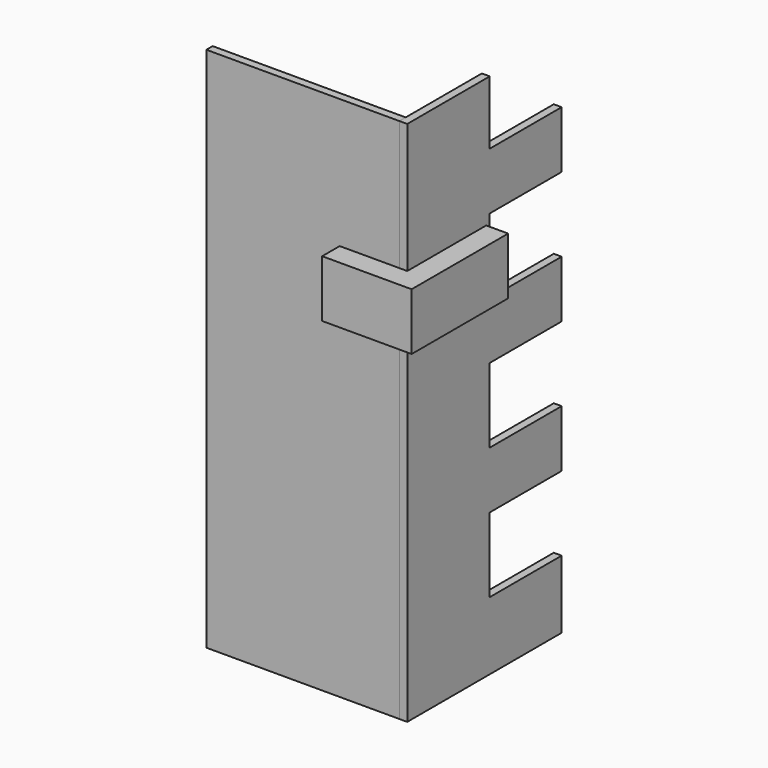
from build123d import *

# Parameters (mm, degrees)
F0_W     = 220
F0_H     = 600
F1_DEPTH = 9
F3_DEPTH = 9
F4_W     = 102.5
F4_H     = 72.5783139467
F4_H_2   = 85
F5_DEPTH = 25
F6_W     = 112.5
F6_H     = 65
F6_W_2   = 25
F7_DEPTH = 25
F8_W     = 25
F8_H     = 65
F9_DEPTH = 77


with BuildPart() as f1:
    # F0 (on Front) → F1 (new body)
    with BuildSketch(Plane.XZ):
        with Locations((-110, 300)):
            Rectangle(F0_W, F0_H)
    extrude(amount=F1_DEPTH)


with BuildPart() as f3:
    # F2 (on Right) → F3 (new body)
    with BuildSketch(Plane.YZ):
        Polygon((-9, 0), (0, 0), (211, 0), (211, 600), (-9, 600), align=None)
    extrude(amount=F3_DEPTH)

    # F4 (on face) → F5 (cut)
    with BuildSketch(Plane.YZ.offset(9)):
        with Locations((159.75, 563.7108430266)):
            Rectangle(F4_W, F4_H)
        with Locations((159.75, 419.9216860533)):
            Rectangle(F4_W, F4_H_2)
        with Locations((159.75, 119.9216860533)):
            Rectangle(F4_W, F4_H_2)
        with Locations((159.75, 269.9216860533)):
            Rectangle(F4_W, F4_H_2)
    extrude(amount=-F5_DEPTH, mode=Mode.SUBTRACT)

    # F6 (on face) → F7 (join)
    with BuildSketch(Plane.YZ.offset(9)):
        with Locations((47.25, 419.9216860533)):
            Rectangle(F6_W, F6_H)
        with Locations((-21.5, 419.9216860533)):
            Rectangle(F6_W_2, F6_H)
    extrude(amount=F7_DEPTH)

    # F8 (on face) → F9 (join)
    with BuildSketch(Plane(origin=(9, 0, 0), x_dir=(0, -1, 0), z_dir=(-1, 0, 0))):
        with Locations((21.5, 419.9216860533)):
            Rectangle(F8_W, F8_H)
    extrude(amount=F9_DEPTH)


solid = Compound([f1.part, f3.part])
